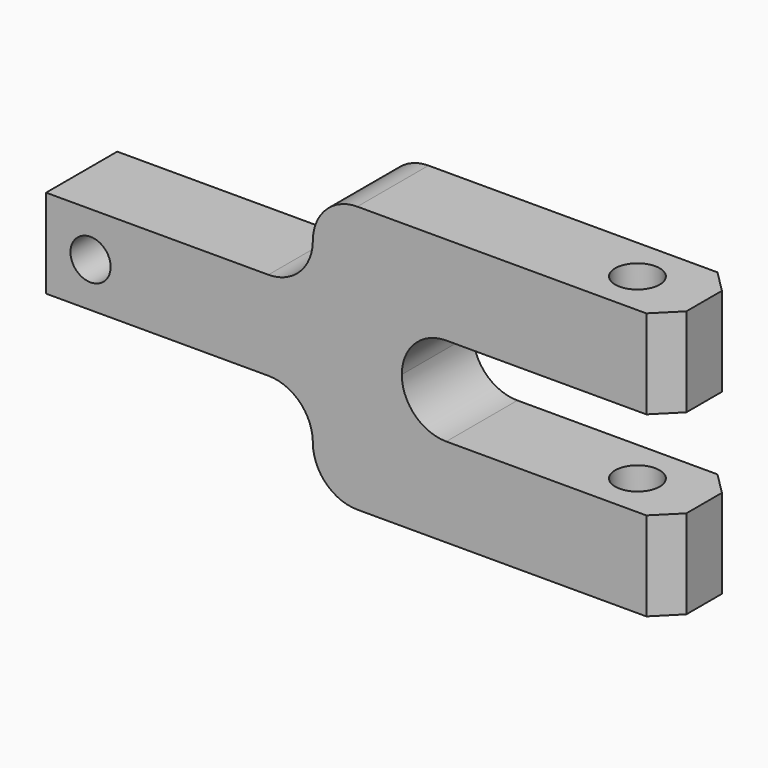
from build123d import *

# Parameters (mm, degrees)
F0_R     = 5.7374218315
F1_DEPTH = 12.7
F2_R     = 12.69999
F3_R     = 12.69999
F4_R     = 12.69999
F5_SIZE2 = 6.35
F5_SIZE  = 6.35
F6_SIZE2 = 6.35
F6_SIZE  = 6.35
F7_R     = 6.35
F8_DEPTH = 127


# Not quite as in the source:
# - a fillet or chamfer is up to 0.001 mm smaller than in the source, because OpenCascade refuses the exact size


with BuildPart() as f1:
    # F0 (on Front) → F1 (new body, symmetric)
    with BuildSketch(Plane.XZ):
        Polygon((26.8901219662, -12.7), (26.8901219662, 12.7), (1.4901219662, 12.7), (-74.7098780338, 12.7), (-74.7098780338, -12.7), (1.4901219662, -12.7), align=None)
        with Locations((-62.0098780338, 0)):
            Circle(F0_R, mode=Mode.SUBTRACT)
        Polygon((1.4901219662, 12.7), (26.8901219662, 12.7), (103.0901219662, 12.7), (103.0901219662, 38.1), (1.4901219662, 38.1), align=None)
        Polygon((103.0901219662, -12.7), (26.8901219662, -12.7), (1.4901219662, -12.7), (1.4901219662, -38.1), (103.0901219662, -38.1), align=None)
    extrude(amount=F1_DEPTH, both=True)

    # F2 (radius 12.7 in the source; OpenCascade refuses exactly that, so slightly less here)
    f2_edges = [f1.edges().sort_by_distance(p)[0] for p in [
        (1.490122, 0, 38.1),
        (1.490122, 0, 12.7),
    ]]
    fillet(f2_edges, radius=F2_R)

    # F3 (radius 12.7 in the source; OpenCascade refuses exactly that, so slightly less here)
    f3_edges = [f1.edges().sort_by_distance(p)[0] for p in [
        (26.890122, 0, 12.7),
        (26.890122, 0, -12.7),
    ]]
    fillet(f3_edges, radius=F3_R)

    # F4 (radius 12.7 in the source; OpenCascade refuses exactly that, so slightly less here)
    f4_edges = [f1.edges().sort_by_distance(p)[0] for p in [
        (1.490122, 0, -12.7),
        (1.490122, 0, -38.1),
    ]]
    fillet(f4_edges, radius=F4_R)

    # F5
    f5_edges = [f1.edges().sort_by_distance(p)[0] for p in [
        (103.090122, -12.7, 25.4),
        (103.090122, 12.7, 25.4),
    ]]
    chamfer(f5_edges, length=F5_SIZE, length2=F5_SIZE2)

    # F6
    f6_edges = [f1.edges().sort_by_distance(p)[0] for p in [
        (103.090122, -12.7, -25.4),
        (103.090122, 12.7, -25.4),
    ]]
    chamfer(f6_edges, length=F6_SIZE, length2=F6_SIZE2)

    # F7 (on Top) → F8 (cut, symmetric)
    with BuildSketch(Plane.XY):
        with Locations((84.0401219662, 0)):
            Circle(F7_R)
    extrude(amount=F8_DEPTH, both=True, mode=Mode.SUBTRACT)


solid = f1.part
